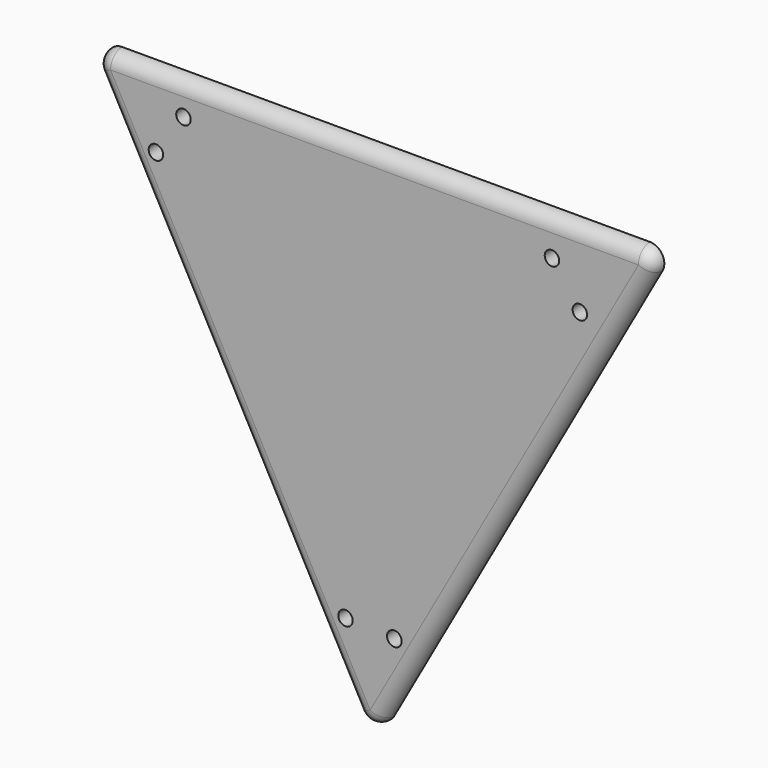
from build123d import *

# Parameters (mm, degrees)
F0_R     = 1.5934819676
F0_R_2   = 1.6180372771
F0_R_3   = 1.5947735427
F0_R_4   = 1.599183997
F0_R_5   = 1.5713503285
F0_R_6   = 1.584959903
F0_R_7   = 1.5945023752
F0_R_8   = 1.5875542678
F1_DEPTH = 3.175
F2_R     = 3.17499


# Not quite as in the source:
# - a fillet or chamfer is up to 0.001 mm smaller than in the source, because OpenCascade refuses the exact size


with BuildPart() as f1:
    # F0 (on Front) → F1 (new body)
    with BuildSketch(Plane.XZ):
        Polygon((64.607411623, 39.6379828453), (-62.5105649233, 39.6379828453), (0, -75.7666006684), align=None)
        with Locations((-5.3829359822, -53.0953221023)):
            Circle(F0_R, mode=Mode.SUBTRACT)
        with Locations((5.3829369135, -53.5846799612)):
            Circle(F0_R_2, mode=Mode.SUBTRACT)
        with Locations((-47.1807047725, 23.7195882946)):
            Circle(F0_R_3, mode=Mode.SUBTRACT)
        with Locations((-41.106056422, 32.5422920287)):
            Circle(F0_R_4, mode=Mode.SUBTRACT)
        with Locations((-6.8510090932, 33.5210077465)):
            Circle(F0_R_5, mode=Mode.SUBTRACT)
        with Locations((7.829724811, 33.5210077465)):
            Circle(F0_R_6, mode=Mode.SUBTRACT)
        with Locations((46.2791621685, 23.0933185667)):
            Circle(F0_R_7, mode=Mode.SUBTRACT)
        with Locations((40.1273407042, 31.5635800362)):
            Circle(F0_R_8, mode=Mode.SUBTRACT)
        with Locations((7.829724811, 33.5210077465)):
            Circle(F0_R_6)
        with Locations((-6.8510090932, 33.5210077465)):
            Circle(F0_R_5)
    extrude(amount=-F1_DEPTH)

    # F2 (radius 3.175 in the source; OpenCascade refuses exactly that, so slightly less here)
    f2_edges = [f1.edges().sort_by_distance(p)[0] for p in [
        (64.607412, 1.5875, 39.637983),
        (-62.510565, 1.5875, 39.637983),
        (0, 1.5875, -75.766601),
        (-31.255282, 0, -18.064309),
        (32.303706, 0, -18.064309),
        (1.048423, 0, 39.637983),
    ]]
    fillet(f2_edges, radius=F2_R)


solid = f1.part
